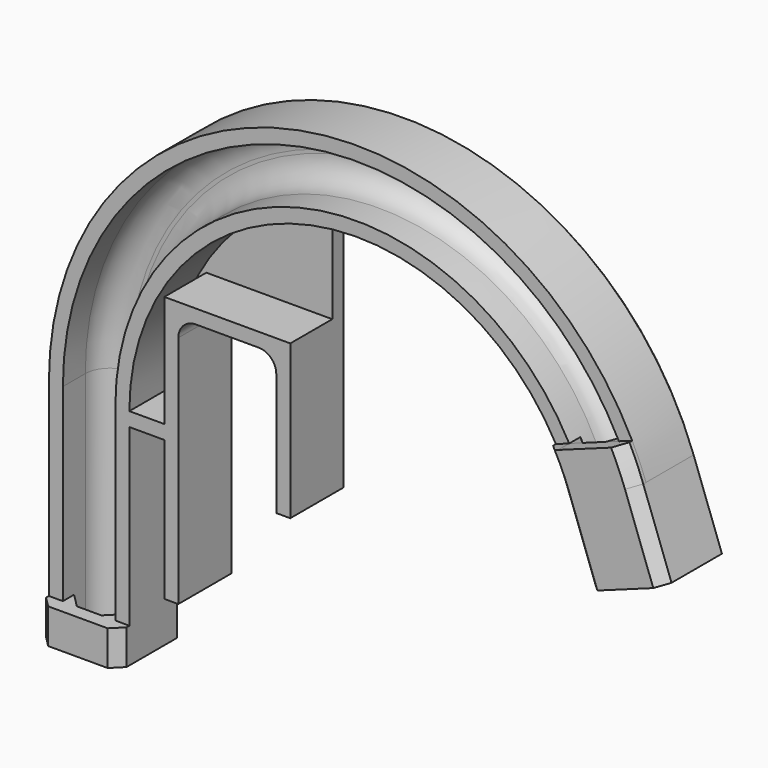
from build123d import *

# Parameters (mm, degrees)
F1_DEPTH     = 4
F2_DEPTH     = 15
F3_R         = 7
F4_SIZE      = 2
F5_W         = 19
F5_H         = 10
F5_W_2       = 4
F6_DEPTH     = 4
F7_T1_DEPTH  = 10
F7_T3_DEPTH  = 23.6580652273
F7_T5_DEPTH  = 23.6580652273
F7_T10_ANGLE = 16.8749432134
F7_T15_ANGLE = 13.853661309
F8_SIZE      = 3
F9_R         = 5


# Not quite as in the source:
# - a fillet or chamfer that OpenCascade refuses, or shapes differently, is made with other operations: its cross-section is extruded or revolved along the edge and cut away or added


with BuildPart() as f1:
    # F0 (on Front) → F1 (new body)
    with BuildSketch(Plane.XZ):
        Polygon((0, 0), (0, 60), (10, 60), (10, 20), (14, 20), (14, 64), (10, 64), (0, 64), (-4, 64), (-4, 0), align=None)
        with BuildLine():
            Line((-19, 0), (-4, 0))
            Line((-4, 0), (-4, 64))
            ThreePointArc((-4, 64), (53.018275741, 131.9517349578), (129.8387908342, 87.5993898895))
            Line((129.8387908342, 87.5993898895), (143.934180146, 92.7296920394))
            ThreePointArc((143.934180146, 92.7296920394), (50.413553076, 146.723851253), (-19, 64))
            Line((-19, 64), (-19, 0))
        make_face()
        with BuildLine():
            ThreePointArc((129.8387908342, 87.5993898895), (53.018275741, 131.9517349578), (-4, 64))
            Line((-4, 64), (0, 64))
            ThreePointArc((0, 64), (12.7505980895, 102.6652298584), (46, 126.1610810717))
            ThreePointArc((46, 126.1610810717), (94.0048047106, 122.1697627956), (126.0800203511, 86.2313093162))
            Line((126.0800203511, 86.2313093162), (129.8387908342, 87.5993898895))
        make_face()
        with BuildLine():
            Line((-23, 0), (-19, 0))
            Line((-19, 0), (-19, 64))
            ThreePointArc((-19, 64), (50.413553076, 146.723851253), (143.934180146, 92.7296920394))
            Line((143.934180146, 92.7296920394), (147.6929506292, 94.0977726127))
            ThreePointArc((147.6929506292, 94.0977726127), (49.7189603653, 150.6630822651), (-23, 64))
            Line((-23, 64), (-23, 0))
        make_face()
        Polygon((10, 64), (14, 64), (14, 92), (42, 92), (42, 52), (46, 52), (46, 92), (46, 96), (10, 96), (10, 92), align=None)
        with BuildLine():
            ThreePointArc((46, 126.1610810717), (12.7505980895, 102.6652298584), (0, 64))
            Line((0, 64), (10, 64))
            Line((10, 64), (10, 92))
            Line((10, 92), (10, 96))
            Line((10, 96), (46, 96))
            Line((46, 96), (46, 126.1610810717))
        make_face()
        Polygon((137.9303256941, 65.3680805733), (129.8387908342, 87.5993898895), (126.0800203511, 86.2313093162), (134.1715552109, 64), align=None)
        Polygon((143.934180146, 92.7296920394), (129.8387908342, 87.5993898895), (137.9303256941, 65.3680805733), (152.0257150059, 70.4983827232), align=None)
        Polygon((147.6929506292, 94.0977726127), (143.934180146, 92.7296920394), (152.0257150059, 70.4983827232), (155.784485489, 71.8664632965), align=None)
    extrude(amount=-F1_DEPTH)

    # F0 (on Front) → F2 (join)
    with BuildSketch(Plane.XZ):
        Polygon((0, 0), (0, 60), (10, 60), (10, 20), (14, 20), (14, 64), (10, 64), (0, 64), (-4, 64), (-4, 0), align=None)
        with BuildLine():
            ThreePointArc((129.8387908342, 87.5993898895), (53.018275741, 131.9517349578), (-4, 64))
            Line((-4, 64), (0, 64))
            ThreePointArc((0, 64), (12.7505980895, 102.6652298584), (46, 126.1610810717))
            ThreePointArc((46, 126.1610810717), (94.0048047106, 122.1697627956), (126.0800203511, 86.2313093162))
            Line((126.0800203511, 86.2313093162), (129.8387908342, 87.5993898895))
        make_face()
        with BuildLine():
            Line((-23, 0), (-19, 0))
            Line((-19, 0), (-19, 64))
            ThreePointArc((-19, 64), (50.413553076, 146.723851253), (143.934180146, 92.7296920394))
            Line((143.934180146, 92.7296920394), (147.6929506292, 94.0977726127))
            ThreePointArc((147.6929506292, 94.0977726127), (49.7189603653, 150.6630822651), (-23, 64))
            Line((-23, 64), (-23, 0))
        make_face()
        Polygon((147.6929506292, 94.0977726127), (143.934180146, 92.7296920394), (152.0257150059, 70.4983827232), (155.784485489, 71.8664632965), align=None)
        Polygon((137.9303256941, 65.3680805733), (129.8387908342, 87.5993898895), (126.0800203511, 86.2313093162), (134.1715552109, 64), align=None)
        Polygon((10, 64), (14, 64), (14, 92), (42, 92), (42, 52), (46, 52), (46, 92), (46, 96), (10, 96), (10, 92), align=None)
    extrude(amount=F2_DEPTH)

    # F3
    f3_edges = [f1.edges().sort_by_distance(p)[0] for p in [
        (50.413553, 0, 146.723851),
        (53.018276, 0, 131.951735),
        (133.884558, 0, 76.483735),
        (147.979948, 0, 81.614037),
        (-19, 0, 32),
        (-4, 0, 32),
    ]]
    fillet(f3_edges, radius=F3_R)

    # F4
    f4_edges = [f1.edges().sort_by_distance(p)[0] for p in [
        (130.125788, 4, 75.115655),
        (151.738718, 4, 82.982118),
        (0, 4, 30),
        (94.004805, 4, 122.169763),
        (49.71896, 4, 150.663082),
        (-23, 4, 32),
    ]]
    chamfer(f4_edges, length=F4_SIZE)

    # F5 (on face) → F6 (join)
    with BuildSketch(Plane.XZ.offset(15)):
        Polygon((137.9303256941, 65.3680805733), (129.8387908342, 87.5993898895), (126.0800203511, 86.2313093162), (134.1715552109, 64), align=None)
        Polygon((147.6929506292, 94.0977726127), (129.8387908342, 87.5993898895), (137.9303256941, 65.3680805733), (155.784485489, 71.8664632965), align=None)
        with Locations((-13.5, 5)):
            Rectangle(F5_W, F5_H)
        with Locations((-2, 5)):
            Rectangle(F5_W_2, F5_H)
        with BuildLine():
            Line((143.7370980696, 103.2997377546), (125.7340390711, 96.7471601534))
            ThreePointArc((125.7340390711, 96.7471601534), (127.95279444, 92.2479321755), (129.8387908342, 87.5993898895))
            Line((129.8387908342, 87.5993898895), (147.6929506292, 94.0977726127))
            ThreePointArc((147.6929506292, 94.0977726127), (145.8460524475, 98.7550831341), (143.7370980696, 103.2997377546))
        make_face()
        with BuildLine():
            ThreePointArc((129.8387908342, 87.5993898895), (127.95279444, 92.2479321755), (125.7340390711, 96.7471601534))
            Line((125.7340390711, 96.7471601534), (121.932649899, 95.3635676459))
            ThreePointArc((121.932649899, 95.3635676459), (124.1827434345, 90.8775534519), (126.0800203511, 86.2313093162))
            Line((126.0800203511, 86.2313093162), (129.8387908342, 87.5993898895))
        make_face()
    extrude(amount=F6_DEPTH)

    # F7: chamfer of 4 on 6 edges, made by hand

    # F7_s2 → F7_t1 (join)
    with BuildSketch(Plane.XY):
        Polygon((-15, -15), (-19, -11), (-19, -15), align=None)
        Polygon((-8, -15), (-4, -11), (-4, -15), align=None)
    extrude(amount=F7_T1_DEPTH)

    # F7_s4 → F7_t3 (join)
    with BuildSketch(Plane(origin=(-12.9656479113, 0, 35.622824865), x_dir=(0, 1, 0), z_dir=(0.3420201433, 0, -0.9396926208))):
        Polygon((-11, 166.9693095239), (-15, 162.9693095239), (-15, 166.9693095239), align=None)
    extrude(amount=F7_T3_DEPTH)

    # F7_s6 → F7_t5 (join)
    with BuildSketch(Plane(origin=(-4.8741130515, 0, 13.3915155488), x_dir=(0, 1, 0), z_dir=(-0.3420201433, 0, 0.9396926208))):
        Polygon((-11, -151.9693095239), (-15, -155.9693095239), (-15, -151.9693095239), align=None)
    extrude(amount=F7_T5_DEPTH)


with BuildPart() as f7_tool8:
    # F7_s9 → F7_t10 (revolve)
    with BuildSketch(Plane(origin=(-12.9656479113, 0, 35.622824865), x_dir=(0, 1, 0), z_dir=(0.3420201433, 0, -0.9396926208))):
        Polygon((-11, 151.9693095239), (-15, 155.9693095239), (-15, 151.9693095239), align=None)
    revolve(axis=Axis((65, -15, 64), (0, -1, 0)), revolution_arc=F7_T10_ANGLE)

    split(bisect_by=Plane(origin=(-16.3858493446, 0, 45.0197510729), x_dir=(0, 1, 0), z_dir=(0.3420201433, 0, -0.9396926208)), keep=Keep.TOP)


with BuildPart() as f1_1:
    add(f1.part)

    # F7_t7: union F7_tool8
    add(f7_tool8.part)


with BuildPart() as f7_tool13:
    # F7_s14 → F7_t15 (revolve)
    with BuildSketch(Plane(origin=(-9.4367447279, 0, 14.0679214359), x_dir=(0, 1, 0), z_dir=(-0.5570736436, 0, 0.830463097))):
        Polygon((-11, -173.6328145012), (-15, -169.6328145012), (-15, -173.6328145012), align=None)
    revolve(axis=Axis((65, -15, 64), (0, 1, 0)), revolution_arc=F7_T15_ANGLE)

    split(bisect_by=Plane(origin=(-16.3858493446, 0, 45.0197510729), x_dir=(0, 1, 0), z_dir=(0.3420201433, 0, -0.9396926208)), keep=Keep.TOP)


with BuildPart() as f1_2:
    add(f1_1.part)

    # F7_t12: union F7_tool13
    add(f7_tool13.part)

    # F8
    f8_edges = [f1_2.edges().sort_by_distance(p)[0] for p in [
        (-23, -19, 5),
        (0, -19, 5),
        (124.182743, -19, 90.877553),
        (145.846052, -19, 98.755083),
        (130.125788, -19, 75.115655),
        (151.738718, -19, 82.982118),
    ]]
    chamfer(f8_edges, length=F8_SIZE)

    # F9
    f9_edges = [f1_2.edges().sort_by_distance(p)[0] for p in [
        (42, -5.5, 92),
        (14, -5.5, 92),
    ]]
    fillet(f9_edges, radius=F9_R)


solid = f1_2.part
